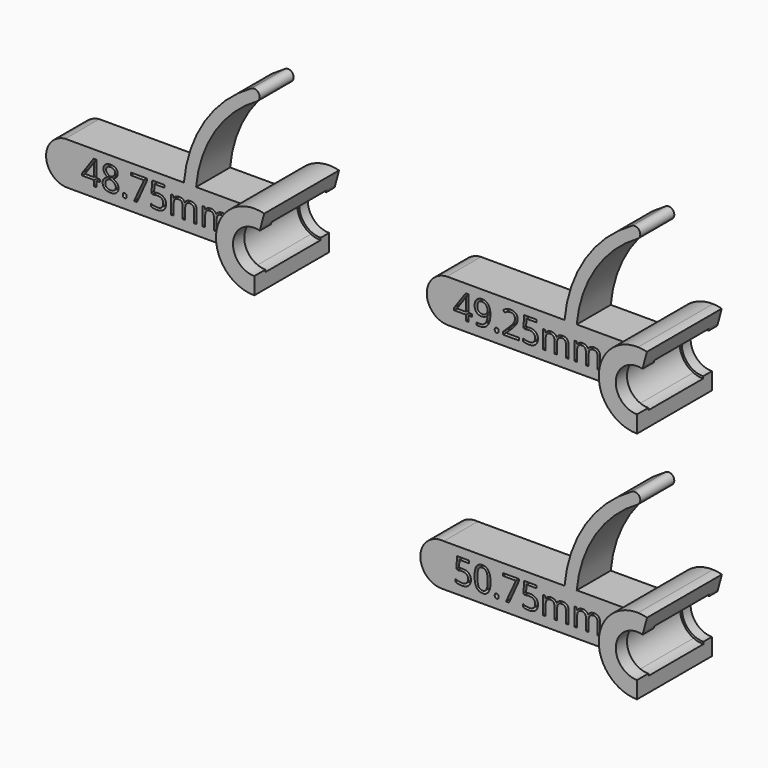
from build123d import *

# Parameters (mm, degrees)
F1_DEPTH       = 6
F1_DEPTH_BACK  = 16
F2_DEPTH       = 10
F3_DEPTH       = 13.4
F3_DEPTH_BACK  = 2.7
F4_TEXT_SIZE   = 7.959916
F5_DEPTH       = 2
F6_DEPTH       = 6
F6_DEPTH_BACK  = 16
F7_DEPTH       = 10
F8_DEPTH       = 13.5
F8_DEPTH_BACK  = 2.7
F9_TEXT_SIZE   = 7.959916
F10_DEPTH      = 2
F11_DEPTH      = 6
F11_DEPTH_BACK = 16
F12_DEPTH      = 10
F13_DEPTH      = 13.5
F13_DEPTH_BACK = 2.7
F14_TEXT_SIZE  = 7.959916
F15_DEPTH      = 2


# Not quite as in the source:
# - Text() gives the source's letters only with a copy of the font that has no kerning and outlines rounded to 1/6400 em; it was checked with that copy


with BuildPart() as f1:
    # F0 (on Front) → F1 (new body, two sides)
    with BuildSketch(Plane.XZ) as f1_sk:
        with BuildLine():
            Line((70, 15), (67.708712, 15))
            ThreePointArc((67.708712, 15), (68.827396, 14.626454), (70, 14.5))
            Line((70, 14.5), (70, 15))
        make_face()
        with BuildLine():
            Line((67.708712, 15), (62.516685, 15))
            ThreePointArc((62.516685, 15), (65.757359, 12.062746), (70, 11))
            Line((70, 11), (70, 14.5))
            ThreePointArc((70, 14.5), (68.827396, 14.626454), (67.708712, 15))
        make_face()
        with BuildLine():
            ThreePointArc((71.415021, 25.314858), (70.836983, 25.435941), (70.249294, 25.494347))
            Line((70.249294, 25.494347), (70.249294, 24.993781))
            ThreePointArc((70.249294, 24.993781), (70.772104, 24.940026), (71.286383, 24.831689))
            Line((71.286383, 24.831689), (71.415021, 25.314858))
        make_face()
        with BuildLine():
            ThreePointArc((70.249294, 25.494347), (68.942206, 25.397321), (67.69519, 24.993781))
            Line((67.69519, 24.993781), (69.750706, 24.993781))
            ThreePointArc((69.750706, 24.993781), (70, 25), (70.249294, 24.993781))
            Line((70.249294, 24.993781), (70.249294, 25.494347))
        make_face()
        with BuildLine():
            ThreePointArc((67.69519, 24.993781), (64.500005, 19.992558), (67.708712, 15))
            Line((67.708712, 15), (70, 15))
            ThreePointArc((70, 15), (65.001555, 19.875314), (69.750706, 24.993781))
            Line((69.750706, 24.993781), (67.69519, 24.993781))
        make_face()
        with BuildLine():
            ThreePointArc((70.249294, 28.996547), (65.864385, 27.99354), (62.512534, 24.993781))
            Line((62.512534, 24.993781), (67.69519, 24.993781))
            ThreePointArc((67.69519, 24.993781), (68.942206, 25.397321), (70.249294, 25.494347))
            Line((70.249294, 25.494347), (70.249294, 28.996547))
        make_face()
        with BuildLine():
            ThreePointArc((72.315489, 28.69704), (71.291106, 28.90691), (70.249294, 28.996547))
            Line((70.249294, 28.996547), (70.249294, 25.494347))
            ThreePointArc((70.249294, 25.494347), (70.836983, 25.435941), (71.415021, 25.314858))
            Line((71.415021, 25.314858), (72.315489, 28.69704))
        make_face()
        with BuildLine():
            ThreePointArc((62.512534, 24.993781), (61.000001, 19.996262), (62.516685, 15))
            Line((62.516685, 15), (67.708712, 15))
            ThreePointArc((67.708712, 15), (64.500005, 19.992558), (67.69519, 24.993781))
            Line((67.69519, 24.993781), (62.512534, 24.993781))
        make_face()
    extrude(amount=F1_DEPTH)
    extrude(f1_sk.sketch, amount=-F1_DEPTH_BACK)

    # F0 (on Front) → F2 (join)
    with BuildSketch(Plane.XZ):
        with BuildLine():
            Line((48.152478, 24.993781), (20.499294, 24.993781))
            ThreePointArc((20.499294, 24.993781), (15.750143, 19.875314), (20.748588, 15))
            Line((20.748588, 15), (62.516685, 15))
            ThreePointArc((62.516685, 15), (61.000001, 19.996262), (62.512534, 24.993781))
            Line((62.512534, 24.993781), (54.512534, 24.993781))
            Line((54.512534, 24.993781), (51.017912, 24.993781))
            Line((51.017912, 24.993781), (48.152478, 24.993781))
        make_face()
        with BuildLine():
            ThreePointArc((64.011169, 49.648646), (53.044344, 39.275005), (48.152478, 24.993781))
            Line((48.152478, 24.993781), (51.017912, 24.993781))
            ThreePointArc((51.017912, 24.993781), (55.469187, 38.006497), (65.443882, 47.474869))
            ThreePointArc((65.443882, 47.474869), (65.74188, 49.230307), (64.011169, 49.648646))
        make_face()
    extrude(amount=-F2_DEPTH)

    # F0 (on Front) → F3 (cut, two sides)
    with BuildSketch(Plane.XZ) as f3_sk:
        with BuildLine():
            ThreePointArc((67.69519, 24.993781), (64.500005, 19.992558), (67.708712, 15))
            Line((67.708712, 15), (70, 15))
            ThreePointArc((70, 15), (65.001555, 19.875314), (69.750706, 24.993781))
            Line((69.750706, 24.993781), (67.69519, 24.993781))
        make_face()
        with BuildLine():
            Line((70, 15), (67.708712, 15))
            ThreePointArc((67.708712, 15), (68.827396, 14.626454), (70, 14.5))
            Line((70, 14.5), (70, 15))
        make_face()
        with BuildLine():
            ThreePointArc((70.249294, 25.494347), (68.942206, 25.397321), (67.69519, 24.993781))
            Line((67.69519, 24.993781), (69.750706, 24.993781))
            ThreePointArc((69.750706, 24.993781), (70, 25), (70.249294, 24.993781))
            Line((70.249294, 24.993781), (70.249294, 25.494347))
        make_face()
        with BuildLine():
            ThreePointArc((71.415021, 25.314858), (70.836983, 25.435941), (70.249294, 25.494347))
            Line((70.249294, 25.494347), (70.249294, 24.993781))
            ThreePointArc((70.249294, 24.993781), (70.772104, 24.940026), (71.286383, 24.831689))
            Line((71.286383, 24.831689), (71.415021, 25.314858))
        make_face()
    extrude(amount=-F3_DEPTH, mode=Mode.SUBTRACT)
    extrude(f3_sk.sketch, amount=F3_DEPTH_BACK, mode=Mode.SUBTRACT)

    # F4 (on face) → F5 (cut)
    with BuildSketch(Plane.XZ):
        with Locations((22.042256, 17.248204)):
            Text('49.25mm', F4_TEXT_SIZE, font='Open Sans', text_align=(TextAlign.LEFT, TextAlign.BOTTOM))
    extrude(amount=-F5_DEPTH, mode=Mode.SUBTRACT)


with BuildPart() as f6:
    # F0 (on Front) → F6 (new body, two sides)
    with BuildSketch(Plane.XZ) as f6_sk:
        with BuildLine():
            ThreePointArc((72.356856, -26.314079), (71.312298, -26.096188), (70.249294, -26.003453))
            Line((70.249294, -26.003453), (69.592539, -29.515114))
            ThreePointArc((69.592539, -29.515114), (70.523933, -29.525012), (71.440301, -29.691937))
            Line((71.440301, -29.691937), (72.356856, -26.314079))
        make_face()
        with BuildLine():
            ThreePointArc((70.249294, -26.003453), (65.854182, -27.011746), (62.499807, -30.025354))
            Line((62.499807, -30.025354), (67.654175, -30.025354))
            ThreePointArc((67.654175, -30.025354), (68.599917, -29.681187), (69.592539, -29.515114))
            Line((69.592539, -29.515114), (70.249294, -26.003453))
        make_face()
        with BuildLine():
            ThreePointArc((62.499807, -30.025354), (61.000013, -35.015229), (62.516685, -40))
            Line((62.516685, -40), (67.708712, -40))
            ThreePointArc((67.708712, -40), (64.500082, -35.030071), (67.654175, -30.025354))
            Line((67.654175, -30.025354), (62.499807, -30.025354))
        make_face()
        with BuildLine():
            Line((67.708712, -40), (62.516685, -40))
            ThreePointArc((62.516685, -40), (65.757359, -42.937254), (70, -44))
            Line((70, -44), (70, -40.5))
            ThreePointArc((70, -40.5), (68.827396, -40.373546), (67.708712, -40))
        make_face()
        with BuildLine():
            Line((70, -40), (67.708712, -40))
            ThreePointArc((67.708712, -40), (68.827396, -40.373546), (70, -40.5))
            Line((70, -40.5), (70, -40))
        make_face()
        with BuildLine():
            ThreePointArc((67.654175, -30.025354), (64.500082, -35.030071), (67.708712, -40))
            Line((67.708712, -40), (70, -40))
            ThreePointArc((70, -40), (65.006342, -35.251763), (69.497113, -30.025354))
            Line((69.497113, -30.025354), (67.654175, -30.025354))
        make_face()
        with BuildLine():
            ThreePointArc((69.592539, -29.515114), (68.599917, -29.681187), (67.654175, -30.025354))
            Line((67.654175, -30.025354), (69.497113, -30.025354))
            Line((69.497113, -30.025354), (69.592539, -29.515114))
        make_face()
        with BuildLine():
            Line((69.592539, -29.515114), (69.497113, -30.025354))
            ThreePointArc((69.497113, -30.025354), (70.410075, -30.016845), (71.309364, -30.174488))
            Line((71.309364, -30.174488), (71.440301, -29.691937))
            ThreePointArc((71.440301, -29.691937), (70.523933, -29.525012), (69.592539, -29.515114))
        make_face()
    extrude(amount=F6_DEPTH)
    extrude(f6_sk.sketch, amount=-F6_DEPTH_BACK)

    # F0 (on Front) → F7 (join)
    with BuildSketch(Plane.XZ):
        with BuildLine():
            Line((48.152478, -30.025354), (19.747113, -30.025354))
            ThreePointArc((19.747113, -30.025354), (14.250568, -34.748237), (19.244226, -40))
            Line((19.244226, -40), (62.516685, -40))
            ThreePointArc((62.516685, -40), (61.000013, -35.015229), (62.499807, -30.025354))
            Line((62.499807, -30.025354), (54.499807, -30.025354))
            Line((54.499807, -30.025354), (51.017912, -30.025354))
            Line((51.017912, -30.025354), (48.152478, -30.025354))
        make_face()
        with BuildLine():
            ThreePointArc((64.011169, -5.370489), (53.044344, -15.74413), (48.152478, -30.025354))
            Line((48.152478, -30.025354), (51.017912, -30.025354))
            ThreePointArc((51.017912, -30.025354), (55.469187, -17.012638), (65.443882, -7.544267))
            ThreePointArc((65.443882, -7.544267), (65.74188, -5.788828), (64.011169, -5.370489))
        make_face()
    extrude(amount=-F7_DEPTH)

    # F0 (on Front) → F8 (cut, two sides)
    with BuildSketch(Plane.XZ) as f8_sk:
        with BuildLine():
            Line((69.592539, -29.515114), (69.497113, -30.025354))
            ThreePointArc((69.497113, -30.025354), (70.410075, -30.016845), (71.309364, -30.174488))
            Line((71.309364, -30.174488), (71.440301, -29.691937))
            ThreePointArc((71.440301, -29.691937), (70.523933, -29.525012), (69.592539, -29.515114))
        make_face()
        with BuildLine():
            ThreePointArc((69.592539, -29.515114), (68.599917, -29.681187), (67.654175, -30.025354))
            Line((67.654175, -30.025354), (69.497113, -30.025354))
            Line((69.497113, -30.025354), (69.592539, -29.515114))
        make_face()
        with BuildLine():
            ThreePointArc((67.654175, -30.025354), (64.500082, -35.030071), (67.708712, -40))
            Line((67.708712, -40), (70, -40))
            ThreePointArc((70, -40), (65.006342, -35.251763), (69.497113, -30.025354))
            Line((69.497113, -30.025354), (67.654175, -30.025354))
        make_face()
        with BuildLine():
            Line((70, -40), (67.708712, -40))
            ThreePointArc((67.708712, -40), (68.827396, -40.373546), (70, -40.5))
            Line((70, -40.5), (70, -40))
        make_face()
    extrude(amount=-F8_DEPTH, mode=Mode.SUBTRACT)
    extrude(f8_sk.sketch, amount=F8_DEPTH_BACK, mode=Mode.SUBTRACT)

    # F9 (on face) → F10 (cut)
    with BuildSketch(Plane.XZ):
        with Locations((22.043814, -37.778094)):
            Text('50.75mm', F9_TEXT_SIZE, font='Open Sans', text_align=(TextAlign.LEFT, TextAlign.BOTTOM))
    extrude(amount=-F10_DEPTH, mode=Mode.SUBTRACT)


with BuildPart() as f11:
    # F0 (on Front) → F11 (new body, two sides)
    with BuildSketch(Plane.XZ) as f11_sk:
        with BuildLine():
            ThreePointArc((-18.576495, 24.664103), (-20.490473, 24.829598), (-22.34461, 24.32673))
            Line((-22.34461, 24.32673), (-20.497189, 24.32673))
            ThreePointArc((-20.497189, 24.32673), (-20, 24.351511), (-19.502811, 24.32673))
            ThreePointArc((-19.502811, 24.32673), (-19.101405, 24.270101), (-18.705905, 24.18114))
            Line((-18.705905, 24.18114), (-18.576495, 24.664103))
        make_face()
        with BuildLine():
            ThreePointArc((-22.34461, 24.32673), (-25.499921, 19.322111), (-22.291288, 14.351511))
            Line((-22.291288, 14.351511), (-20, 14.351511))
            ThreePointArc((-20, 14.351511), (-24.993801, 19.102608), (-20.497189, 24.32673))
            Line((-20.497189, 24.32673), (-22.34461, 24.32673))
        make_face()
        with BuildLine():
            Line((-20, 14.351511), (-22.291288, 14.351511))
            ThreePointArc((-22.291288, 14.351511), (-21.172604, 13.977964), (-20, 13.851511))
            Line((-20, 13.851511), (-20, 14.351511))
        make_face()
        with BuildLine():
            Line((-22.291288, 14.351511), (-27.483315, 14.351511))
            ThreePointArc((-27.483315, 14.351511), (-24.242641, 11.414257), (-20, 10.351511))
            Line((-20, 10.351511), (-20, 13.851511))
            ThreePointArc((-20, 13.851511), (-21.172604, 13.977964), (-22.291288, 14.351511))
        make_face()
        with BuildLine():
            ThreePointArc((-27.499813, 24.32673), (-28.999988, 19.336625), (-27.483315, 14.351511))
            Line((-27.483315, 14.351511), (-22.291288, 14.351511))
            ThreePointArc((-22.291288, 14.351511), (-25.499921, 19.322111), (-22.34461, 24.32673))
            Line((-22.34461, 24.32673), (-27.499813, 24.32673))
        make_face()
        with BuildLine():
            ThreePointArc((-17.670629, 28.044843), (-23.184252, 27.769381), (-27.499813, 24.32673))
            Line((-27.499813, 24.32673), (-22.34461, 24.32673))
            ThreePointArc((-22.34461, 24.32673), (-20.490473, 24.829598), (-18.576495, 24.664103))
            Line((-18.576495, 24.664103), (-17.670629, 28.044843))
        make_face()
    extrude(amount=F11_DEPTH)
    extrude(f11_sk.sketch, amount=-F11_DEPTH_BACK)

    # F0 (on Front) → F12 (join)
    with BuildSketch(Plane.XZ):
        with BuildLine():
            Line((-41.351733, 24.32673), (-69.252811, 24.32673))
            ThreePointArc((-69.252811, 24.32673), (-73.749424, 19.102608), (-68.755623, 14.351511))
            Line((-68.755623, 14.351511), (-27.483315, 14.351511))
            ThreePointArc((-27.483315, 14.351511), (-28.999988, 19.336625), (-27.499813, 24.32673))
            Line((-27.499813, 24.32673), (-35.499813, 24.32673))
            Line((-35.499813, 24.32673), (-38.486299, 24.32673))
            Line((-38.486299, 24.32673), (-41.351733, 24.32673))
        make_face()
        with BuildLine():
            ThreePointArc((-25.493042, 48.981595), (-36.459867, 38.607953), (-41.351733, 24.32673))
            Line((-41.351733, 24.32673), (-38.486299, 24.32673))
            ThreePointArc((-38.486299, 24.32673), (-34.035025, 37.339445), (-24.060329, 46.807817))
            ThreePointArc((-24.060329, 46.807817), (-23.762331, 48.563256), (-25.493042, 48.981595))
        make_face()
    extrude(amount=-F12_DEPTH)

    # F0 (on Front) → F13 (cut, two sides)
    with BuildSketch(Plane.XZ) as f13_sk:
        with BuildLine():
            Line((-20, 14.351511), (-22.291288, 14.351511))
            ThreePointArc((-22.291288, 14.351511), (-21.172604, 13.977964), (-20, 13.851511))
            Line((-20, 13.851511), (-20, 14.351511))
        make_face()
        with BuildLine():
            ThreePointArc((-22.34461, 24.32673), (-25.499921, 19.322111), (-22.291288, 14.351511))
            Line((-22.291288, 14.351511), (-20, 14.351511))
            ThreePointArc((-20, 14.351511), (-24.993801, 19.102608), (-20.497189, 24.32673))
            Line((-20.497189, 24.32673), (-22.34461, 24.32673))
        make_face()
        with BuildLine():
            ThreePointArc((-18.576495, 24.664103), (-20.490473, 24.829598), (-22.34461, 24.32673))
            Line((-22.34461, 24.32673), (-20.497189, 24.32673))
            ThreePointArc((-20.497189, 24.32673), (-20, 24.351511), (-19.502811, 24.32673))
            ThreePointArc((-19.502811, 24.32673), (-19.101405, 24.270101), (-18.705905, 24.18114))
            Line((-18.705905, 24.18114), (-18.576495, 24.664103))
        make_face()
    extrude(amount=-F13_DEPTH, mode=Mode.SUBTRACT)
    extrude(f13_sk.sketch, amount=F13_DEPTH_BACK, mode=Mode.SUBTRACT)

    # F14 (on face) → F15 (cut)
    with BuildSketch(Plane.XZ):
        with Locations((-65.417305, 16.680252)):
            Text('48.75mm', F14_TEXT_SIZE, font='Open Sans', text_align=(TextAlign.LEFT, TextAlign.BOTTOM))
    extrude(amount=-F15_DEPTH, mode=Mode.SUBTRACT)


solid = Compound([f1.part, f6.part, f11.part])
